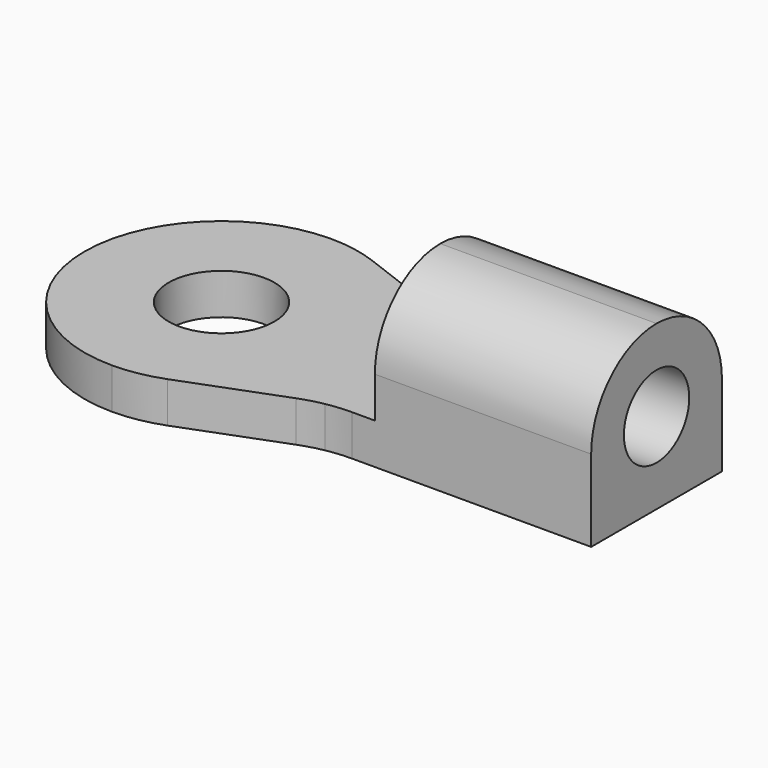
from build123d import *

# Parameters (mm, degrees)
F0_R     = 1.1
F1_DEPTH = 0.85
F2_W     = 4.5
F2_H     = 3.4
F3_DEPTH = 2.55
F4_R     = 1.69999
F5_R     = 0.85
F6_DEPTH = 25


# Not quite as in the source:
# - a fillet or chamfer is up to 0.001 mm smaller than in the source, because OpenCascade refuses the exact size


with BuildPart() as f1:
    # F0 (on Top) → F1 (new body)
    with BuildSketch(Plane.XY):
        with BuildLine():
            Line((6.9231632929, 1.15), (11.9, 1.15))
            Line((11.9, 1.15), (11.9, 4.55))
            Line((11.9, 4.55), (6.9231632929, 4.55))
            ThreePointArc((6.9231632929, 4.55), (6.6604632751, 4.5621330721), (6.4, 4.598428982))
            ThreePointArc((6.4, 4.598428982), (6.1524055327, 4.656201087), (5.9109449246, 4.7358089455))
            Line((5.9109449246, 4.7358089455), (3.8622183683, 5.5141910545))
            ThreePointArc((3.8622183683, 5.5141910545), (3.3645655909, 5.6531629016), (2.85, 5.7))
            ThreePointArc((2.85, 5.7), (0.8347456736, 4.8652543264), (0, 2.85))
            ThreePointArc((0, 2.85), (0.8347456736, 0.8347456736), (2.85, 0))
            ThreePointArc((2.85, 0), (3.3645655909, 0.0468370984), (3.8622183683, 0.1858089455))
            Line((3.8622183683, 0.1858089455), (5.9109449246, 0.9641910545))
            ThreePointArc((5.9109449246, 0.9641910545), (6.1524055327, 1.043798913), (6.4, 1.101571018))
            ThreePointArc((6.4, 1.101571018), (6.6604632751, 1.1378669279), (6.9231632929, 1.15))
        make_face()
        with Locations((2.85, 2.85)):
            Circle(F0_R, mode=Mode.SUBTRACT)
    extrude(amount=F1_DEPTH)

    # F2 (on face) → F3 (join)
    with BuildSketch(Plane.XY.offset(0.85)):
        with Locations((9.65, 2.85)):
            Rectangle(F2_W, F2_H)
    extrude(amount=F3_DEPTH)

    # F4 (radius 1.7 in the source; OpenCascade refuses exactly that, so slightly less here)
    f4_edges = [f1.edges().sort_by_distance(p)[0] for p in [
        (9.65, 4.55, 3.4),
        (9.65, 1.15, 3.4),
    ]]
    fillet(f4_edges, radius=F4_R)

    # F5 (on face) → F6 (cut)
    with BuildSketch(Plane.YZ.offset(11.9)):
        with Locations((2.85, 1.7)):
            Circle(F5_R)
    extrude(amount=-F6_DEPTH, mode=Mode.SUBTRACT)


solid = f1.part
